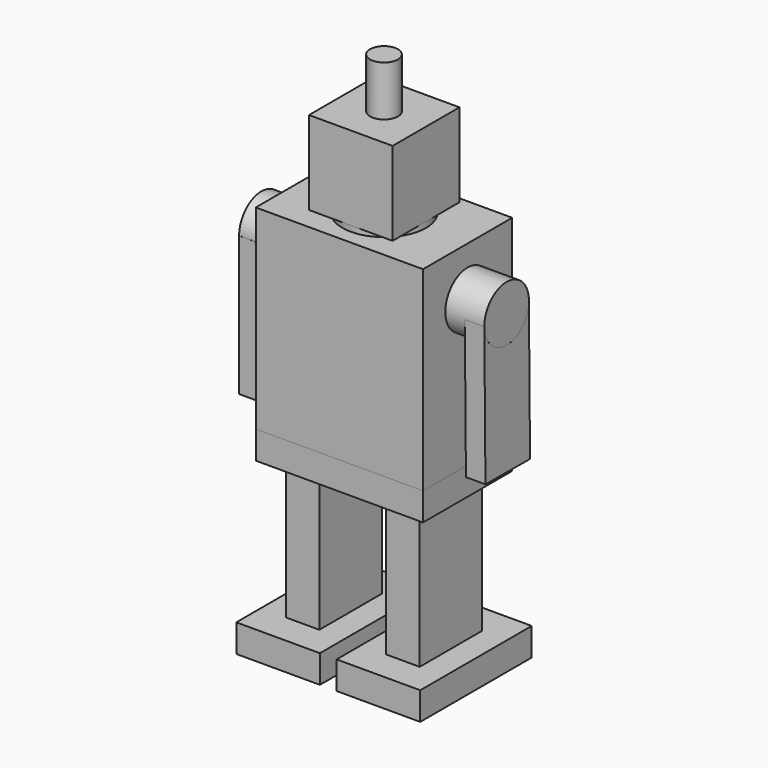
from build123d import *

# Parameters (mm, degrees)
F0_W          = 76.2
F0_H          = 114.3
F1_DEPTH      = 50.8
F2_R          = 12.7
F3_DEPTH      = 76.2
F4_W          = 76.2
F4_H          = 50.8
F4_R          = 12.7
F5_DEPTH      = 25.4
F6_R          = 12.7
F7_DEPTH      = 38.1
F8_R          = 12.7
F9_DEPTH      = 17.78
F9_DEPTH_BACK = 93.98
F11_DEPTH     = 8.89
F12_W         = 25.4
F12_H         = 63.5
F13_DEPTH     = 8.89
F14_W         = 76.2
F14_H         = 50.8
F15_DEPTH     = 12.7
F16_W         = 15.24
F16_H         = 35.56
F17_DEPTH     = 63.5
F18_W         = 38.1
F18_H         = 63.5
F18_W_2       = 15.24
F18_H_2       = 35.56
F19_DEPTH     = 12.7
F20_R         = 19.05
F21_DEPTH     = 2.54
F22_W         = 38.1
F22_H         = 38.1
F23_DEPTH     = 38.1
F24_R         = 6.35
F25_DEPTH     = 40.64
F26_R         = 6.35
F27_DEPTH     = 63.5
F28_R         = 12.7
F29_DEPTH     = 38.1


# Not quite as in the source:
# - a feature of the source that left no trace in its solid (it failed there, or was rolled back) is left out


with BuildPart() as f1:
    # F0 (on Front) → F1 (new body)
    with BuildSketch(Plane.XZ):
        Rectangle(F0_W, F0_H)
    extrude(amount=F1_DEPTH)

    # F2 (on face) → F3 (cut)
    with BuildSketch(Plane.YZ.offset(38.1)):
        with Locations((-25.4, 34.8205566406)):
            Circle(F2_R)
    extrude(amount=-F3_DEPTH, mode=Mode.SUBTRACT)

    # F4 (on face) → F5 (cut)
    with BuildSketch(Plane(origin=(0, 0, -57.15), x_dir=(1, 0, 0), z_dir=(0, 0, -1))):
        with Locations((0, 25.4)):
            Rectangle(F4_W, F4_H)
        with Locations((0, 25.4)):
            Circle(F4_R, mode=Mode.SUBTRACT)
        with Locations((0, 25.4)):
            Circle(F4_R)
    extrude(amount=-F5_DEPTH, mode=Mode.SUBTRACT)

    # F6 (on face) → F7 (cut)
    with BuildSketch(Plane(origin=(0, 0, -31.75), x_dir=(1, 0, 0), z_dir=(0, 0, -1))):
        with Locations((0, 25.4)):
            Circle(F6_R)
    extrude(amount=-F7_DEPTH, mode=Mode.SUBTRACT)


with BuildPart() as f9:
    # F8 (on face) → F9 (new body, two sides)
    with BuildSketch(Plane.YZ.offset(38.1)) as f9_sk:
        with Locations((-25.4, 34.8205566406)):
            Circle(F8_R)
    extrude(amount=F9_DEPTH)
    extrude(f9_sk.sketch, amount=-F9_DEPTH_BACK)


with BuildPart() as f11:
    # F10 (on face) → F11 (new body)
    with BuildSketch(Plane.YZ.offset(55.88)):
        with BuildLine():
            ThreePointArc((-12.7027346591, 34.5570175282), (-25.4681418528, 22.1207394495), (-38.0993622657, 34.6932851007))
            Line((-38.0993622657, 34.6932851007), (-37.4630045663, -28.8035262277))
            Line((-37.4630045663, -28.8035262277), (-12.0663769597, -28.9397938002))
            Line((-12.0663769597, -28.9397938002), (-12.7027346591, 34.5570175282))
        make_face()
    extrude(amount=-F11_DEPTH)


with BuildPart() as f13:
    # F12 (on face) → F13 (new body)
    with BuildSketch(Plane(origin=(-55.88, 0, 0), x_dir=(0, -1, 0), z_dir=(-1, 0, 0))):
        with Locations((25.4000125671, 3.0884229026)):
            Rectangle(F12_W, F12_H)
    extrude(amount=-F13_DEPTH)


with BuildPart() as f15:
    # F14 (on face) → F15 (new body)
    with BuildSketch(Plane(origin=(0, 0, -31.75), x_dir=(1, 0, 0), z_dir=(0, 0, -1))):
        with Locations((0, 25.4)):
            Rectangle(F14_W, F14_H)
    extrude(amount=F15_DEPTH)


with BuildPart() as f17:
    # F16 (on face) → F17 (new body)
    with BuildSketch(Plane(origin=(0, 0, -44.45), x_dir=(1, 0, 0), z_dir=(0, 0, -1))):
        with Locations((-22.86, 25.4)):
            Rectangle(F16_W, F16_H)
    extrude(amount=F17_DEPTH)


with BuildPart() as f17b:
    # F16 (on face) → F17, piece 2 (new body)
    with BuildSketch(Plane(origin=(0, 0, -44.45), x_dir=(1, 0, 0), z_dir=(0, 0, -1))):
        with Locations((22.86, 25.4)):
            Rectangle(F16_W, F16_H)
    extrude(amount=F17_DEPTH)


with BuildPart() as f19:
    # F18 (on face) → F19 (new body)
    with BuildSketch(Plane(origin=(0, 0, -107.95), x_dir=(1, 0, 0), z_dir=(0, 0, -1))):
        with Locations((-22.86, 25.4)):
            Rectangle(F18_W, F18_H)
        with Locations((-22.86, 25.4)):
            Rectangle(F18_W_2, F18_H_2, mode=Mode.SUBTRACT)
        with Locations((-22.86, 25.4)):
            Rectangle(F18_W_2, F18_H_2)
    extrude(amount=F19_DEPTH)


with BuildPart() as f19b:
    # F18 (on face) → F19, piece 2 (new body)
    with BuildSketch(Plane(origin=(0, 0, -107.95), x_dir=(1, 0, 0), z_dir=(0, 0, -1))):
        with Locations((22.86, 25.4)):
            Rectangle(F18_W, F18_H)
    extrude(amount=F19_DEPTH)


with BuildPart() as f21:
    # F20 (on face) → F21 (new body)
    with BuildSketch(Plane.XY.offset(57.15)):
        with Locations((0, -25.266315788)):
            Circle(F20_R)
    extrude(amount=F21_DEPTH)


with BuildPart() as f23:
    # F22 (on face) → F23 (new body)
    with BuildSketch(Plane.XY.offset(59.69)):
        with Locations((0, -25.266315788)):
            Rectangle(F22_W, F22_H)
    extrude(amount=F23_DEPTH)


with BuildPart() as f25_tool:
    # F24 (on face) → F25 (new body)
    with BuildSketch(Plane.XY.offset(97.79)):
        with Locations((0, -25.266315788)):
            Circle(F24_R)
    extrude(amount=-F25_DEPTH)


with BuildPart() as f21_1:
    add(f21.part)

    # F25: cut by f25_tool
    add(f25_tool.part, mode=Mode.SUBTRACT)


with BuildPart() as f23_1:
    add(f23.part)

    # F25: cut by f25_tool
    add(f25_tool.part, mode=Mode.SUBTRACT)


with BuildPart() as f27:
    # F26 (on face) → F27 (new body)
    with BuildSketch(Plane.XY.offset(57.15)):
        with Locations((0, -25.4)):
            Circle(F26_R)
    extrude(amount=F27_DEPTH)


with BuildPart() as f29:
    # F28 (on face) → F29 (new body)
    with BuildSketch(Plane.XY.offset(-31.75)):
        with Locations((0, -25.4)):
            Circle(F28_R)
    extrude(amount=F29_DEPTH)


solid = Compound([f1.part, f9.part, f11.part, f13.part, f15.part, f17.part, f17b.part, f19.part, f19b.part, f21_1.part, f23_1.part, f27.part, f29.part])
